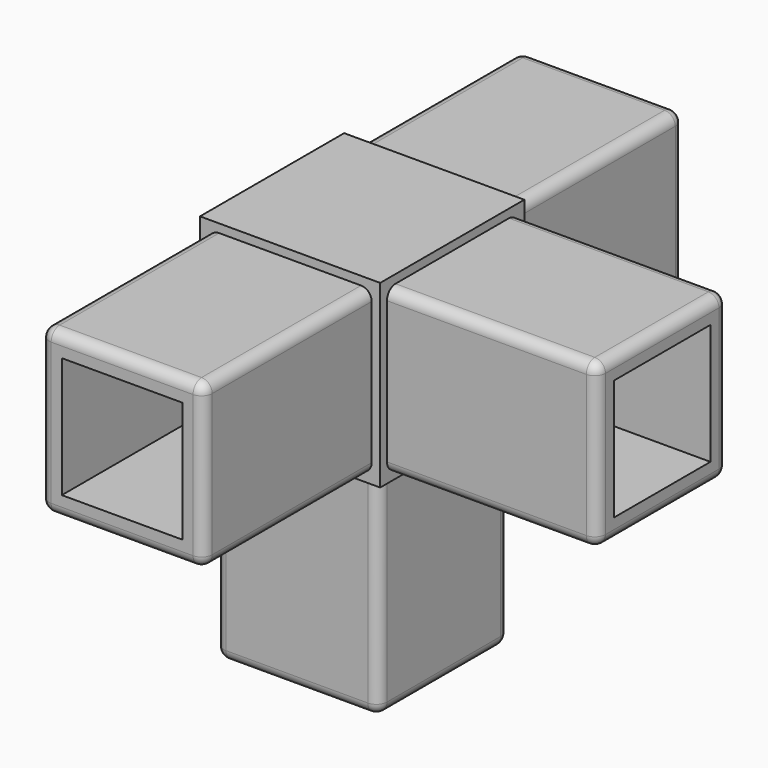
from build123d import *

# Parameters (mm, degrees)
F0_W            = 25.4
F0_H            = 25.4
F1_DEPTH        = 12.7
F2_W            = 23
F2_H            = 23
F2_W_2          = 17
F2_H_2          = 17
F3_DEPTH        = 29.6
F3_COPIES_COUNT = 3
F3_COPIES_ANGLE = 180
F4_R            = 1.5


# Not quite as in the source:
# - a pattern or mirror of a feature is missing from the dataset's text; its kind, count and spacing are read off the source's solid


with BuildPart() as f1:
    # F0 (on Front) → F1 (new body, symmetric)
    with BuildSketch(Plane.XZ):
        Rectangle(F0_W, F0_H)
    extrude(amount=F1_DEPTH, both=True)

    # F2 (on face) → F3 (join)
    with BuildSketch(Plane.XZ.offset(12.7)):
        Rectangle(F2_W, F2_H)
        Rectangle(F2_W_2, F2_H_2, mode=Mode.SUBTRACT)
    f3 = extrude(amount=F3_DEPTH)

    # F3_copies: F3 ×3 about axis
    f3_copies_axis = Axis((0, 0, 0), (0, 0, 1))
    for i in range(1, F3_COPIES_COUNT):
        add(f3.rotate(f3_copies_axis, i * F3_COPIES_ANGLE / (F3_COPIES_COUNT - 1)))

    # F3_copies1: F3 across plane
    add(f3.mirror(Plane(origin=(0, 0, 0), x_dir=(0, -0.7071067812, -0.7071067812), z_dir=(0, 0.7071067812, -0.7071067812))))

    # F4
    f4_edges = [f1.edges().sort_by_distance(p)[0] for p in [
        (11.5, -27.5, 11.5),
        (11.5, -27.5, -11.5),
        (-11.5, -27.5, 11.5),
        (-11.5, -27.5, -11.5),
        (0, -42.3, 11.5),
        (11.5, -42.3, 0),
        (0, -42.3, -11.5),
        (-11.5, -42.3, 0),
        (-11.5, 27.5, -11.5),
        (-11.5, 27.5, 11.5),
        (-11.5, 42.3, 0),
        (11.5, 27.5, -11.5),
        (0, 42.3, -11.5),
        (11.5, 27.5, 11.5),
        (11.5, 42.3, 0),
        (0, 42.3, 11.5),
        (27.5, 11.5, 11.5),
        (27.5, -11.5, 11.5),
        (42.3, 0, 11.5),
        (27.5, -11.5, -11.5),
        (42.3, -11.5, 0),
        (27.5, 11.5, -11.5),
        (42.3, 0, -11.5),
        (42.3, 11.5, 0),
        (11.5, -11.5, -27.5),
        (11.5, 11.5, -27.5),
        (11.5, 0, -42.3),
        (-11.5, -11.5, -27.5),
        (0, -11.5, -42.3),
        (-11.5, 11.5, -27.5),
        (-11.5, 0, -42.3),
        (0, 11.5, -42.3),
    ]]
    fillet(f4_edges, radius=F4_R)


solid = f1.part
